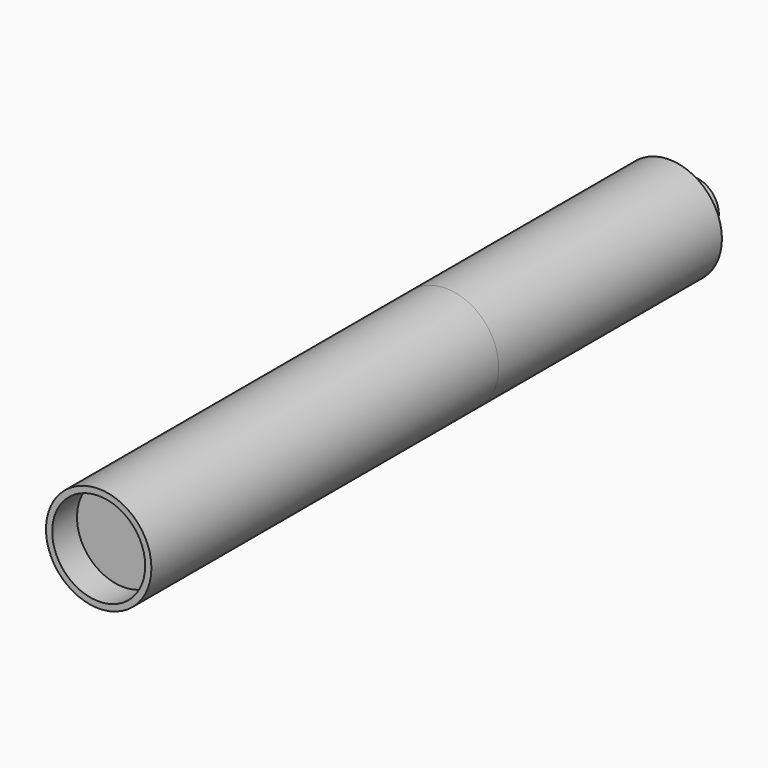
from build123d import *

# Parameters (mm, degrees)
F0_R          = 8.5
F1_DEPTH      = 90
F2_R          = 8.5
F3_DEPTH      = 20
F3_DEPTH_BACK = 25
F4_R          = 4
F5_DEPTH      = 5
F6_R          = 8.45
F7_DEPTH      = 20
F8_DEPTH      = 20
F10_R         = 7.5
F11_DEPTH     = 5


# Not quite as in the source:
# - the program builds the solid bodies; features that only make, move or delete a surface that nothing else refers to are left out


with BuildPart() as f1:
    # F0 (on Front) → F1 (new body)
    with BuildSketch(Plane.XZ):
        Circle(F0_R)
    extrude(amount=F1_DEPTH)

    # F10 (on face) → F11 (cut)
    with BuildSketch(Plane.XZ.offset(90)):
        Circle(F10_R)
    extrude(amount=-F11_DEPTH, mode=Mode.SUBTRACT)


with BuildPart() as f3:
    # F2 (on Front) → F3 (new body, two sides)
    with BuildSketch(Plane.XZ) as f3_sk:
        Circle(F2_R)
    extrude(amount=F3_DEPTH)
    extrude(f3_sk.sketch, amount=-F3_DEPTH_BACK)

    # F6 (on face) → F7 (cut)
    with BuildSketch(Plane(origin=(0, 25, 0), x_dir=(-1, 0, 0), z_dir=(0, 1, 0))):
        Circle(F6_R)
    extrude(amount=-F7_DEPTH, mode=Mode.SUBTRACT)


with BuildPart() as f5:
    # F4 (on face) → F5 (new body)
    with BuildSketch(Plane(origin=(0, 25, 0), x_dir=(-1, 0, 0), z_dir=(0, 1, 0))):
        Circle(F4_R)
    extrude(amount=F5_DEPTH)


with BuildPart() as f8:
    # F4 (on face) → F8 (new body)
    with BuildSketch(Plane(origin=(0, 25, 0), x_dir=(-1, 0, 0), z_dir=(0, 1, 0))):
        Circle(F4_R)
    extrude(amount=-F8_DEPTH)


solid = Compound([f1.part, f3.part, f5.part, f8.part])
